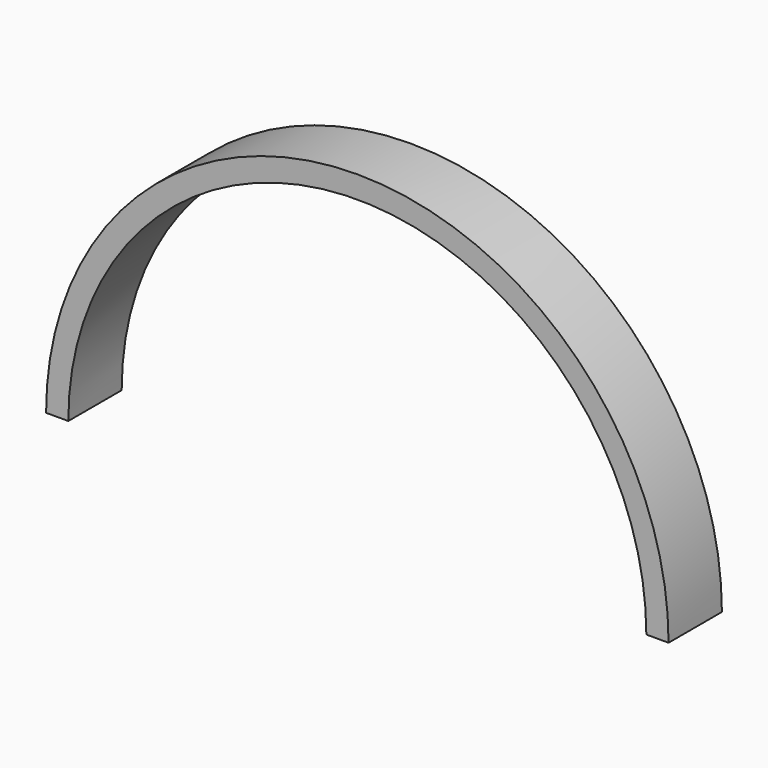
from build123d import *

# Parameters (mm, degrees)
F1_DEPTH = 38.1


with BuildPart() as f1:
    # F0 (on Front) → F1 (new body)
    with BuildSketch(Plane.XZ):
        with BuildLine():
            Line((165.1, 0), (177.8, 0))
            ThreePointArc((177.8, 0), (0, 177.8), (-177.8, 0))
            Line((-177.8, 0), (-165.1, 0))
            ThreePointArc((-165.1, 0), (0, 165.1), (165.1, 0))
        make_face()
    extrude(amount=F1_DEPTH)


solid = f1.part
